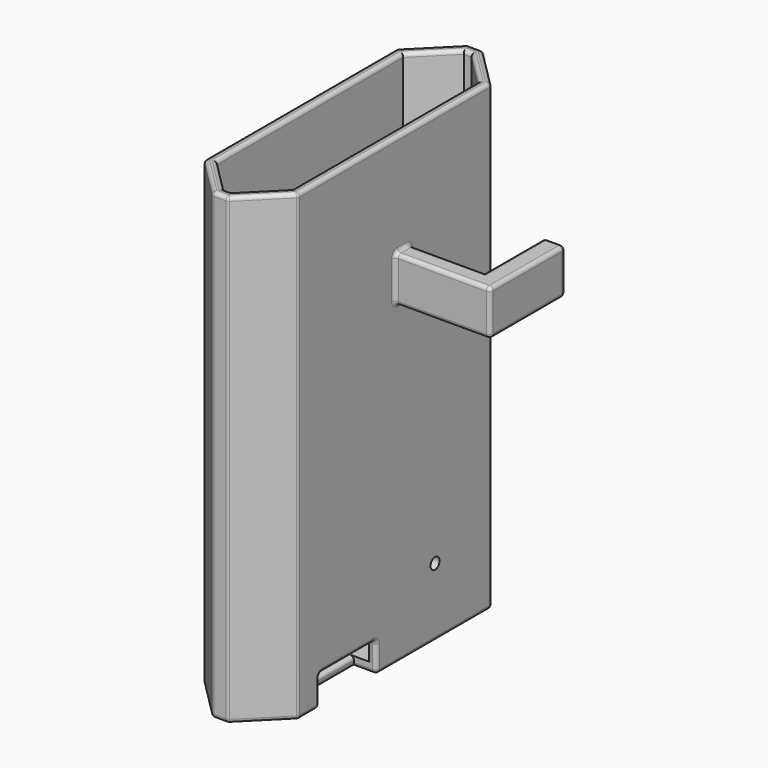
from build123d import *

# Parameters (mm, degrees)
F1_DEPTH = 2.5
F2_DEPTH = 123.5
F3_W     = 6
F3_H     = 19
F4_DEPTH = 8
F6_D     = 3
F6_DEPTH = 5
F6_TIP   = 0.9012909285
F5_W     = 5
F5_H     = 12
F7_DEPTH = 25.5
F8_START = 20
F5_W_2   = 20
F8_DEPTH = 5.5
F9_R     = 1


with BuildPart() as f1:
    # F0 (on Top) → F1 (new body)
    with BuildSketch(Plane.XY):
        Polygon((10, 31), (1, 40), (-1, 40), (-10, 31), (-10, -31), (-1, -40), (1, -40), (10, -31), align=None)
    extrude(amount=F1_DEPTH)

    # F0 (on Top) → F2 (join)
    with BuildSketch(Plane.XY):
        Polygon((12.500000447, -32.0355340911), (12.500000447, 32.0355340911), (2.0355340911, 42.500000447), (-2.0355340911, 42.500000447), (-12.500000447, 32.0355340911), (-12.500000447, -32.0355340911), (-2.0355340911, -42.500000447), (2.0355340911, -42.500000447), align=None)
        Polygon((-1, 40), (1, 40), (10, 31), (10, -31), (1, -40), (-1, -40), (-10, -31), (-10, 31), align=None, mode=Mode.SUBTRACT)
    extrude(amount=F2_DEPTH)

    # F3 (on face) → F4 (cut)
    with BuildSketch(Plane(origin=(0, 0, 0), x_dir=(1, 0, 0), z_dir=(0, 0, -1))):
        with Locations((9.500000447, 15.5355340911)):
            Rectangle(F3_W, F3_H)
    extrude(amount=-F4_DEPTH, mode=Mode.SUBTRACT)

    # F6
    with Locations(Plane.YZ.offset(12.500000447)):
        with Locations((13.5, 18.25)):
            Hole(F6_D / 2, depth=F6_DEPTH)
            with Locations((0, 0, -(F6_DEPTH + F6_TIP / 2))):  # 118° drill point
                Cone(0, F6_D / 2, F6_TIP, mode=Mode.SUBTRACT)

    # F5 (on face) → F7 (join)
    with BuildSketch(Plane.YZ.offset(12.500000447)):
        with Locations((2.5, 90.5)):
            Rectangle(F5_W, F5_H)
    extrude(amount=F7_DEPTH)

    # F5 (on face) → F8 (join)
    with BuildSketch(Plane.YZ.offset(12.500000447).offset(F8_START)):
        with Locations((15, 90.5)):
            Rectangle(F5_W_2, F5_H)
    extrude(amount=F8_DEPTH)

    # F9
    f9_edges = [f1.edges().sort_by_distance(p)[0] for p in [
        (12.5, 0, 123.5),
        (7.267767, 37.267767, 123.5),
        (0, 42.5, 123.5),
        (-7.267767, 37.267767, 123.5),
        (-12.5, 0, 123.5),
        (-7.267767, -37.267767, 123.5),
        (0, -42.5, 123.5),
        (7.267767, -37.267767, 123.5),
        (0, 40, 123.5),
        (5.5, 35.5, 123.5),
        (10, 0, 123.5),
        (5.5, -35.5, 123.5),
        (0, -40, 123.5),
        (-5.5, -35.5, 123.5),
        (-10, 0, 123.5),
        (-5.5, 35.5, 123.5),
        (22.5, 5, 96.5),
        (32.5, 15, 96.5),
        (35.25, 25, 96.5),
        (38, 12.5, 96.5),
        (25.25, 0, 96.5),
        (12.5, 2.5, 96.5),
        (25.25, 0, 84.5),
        (38, 12.5, 84.5),
        (35.25, 25, 84.5),
        (32.5, 15, 84.5),
        (22.5, 5, 84.5),
        (12.5, 2.5, 84.5),
        (7.267767, -37.267767, 0),
        (0, -42.5, 0),
        (-7.267767, -37.267767, 0),
        (-12.5, 0, 0),
        (-7.267767, 37.267767, 0),
        (0, 42.5, 0),
        (7.267767, 37.267767, 0),
        (12.5, 13, 0),
        (9.5, -6.035534, 0),
        (6.5, -15.535534, 0),
        (9.5, -25.035534, 0),
        (12.5, -28.535534, 0),
        (-2.035534, 42.5, 61.75),
        (-12.5, 32.035534, 61.75),
        (-12.5, -32.035534, 61.75),
        (-2.035534, -42.5, 61.75),
        (2.035534, 42.5, 61.75),
        (12.5, 32.035534, 61.75),
        (12.5, -32.035534, 61.75),
        (2.035534, -42.5, 61.75),
        (11.25, -6.035534, 8),
        (10, -15.535534, 8),
        (11.25, -25.035534, 8),
        (12.5, -15.535534, 8),
        (6.5, -15.535534, 2.5),
        (32.5, 25, 90.5),
        (38, 25, 90.5),
        (38, 0, 90.5),
        (10, -25.035534, 5.25),
        (12.5, -25.035534, 4),
        (10, -6.035534, 5.25),
        (12.5, -6.035534, 4),
        (12.5, 5, 90.5),
        (12.5, 0, 90.5),
    ]]
    fillet(f9_edges, radius=F9_R)


solid = f1.part
